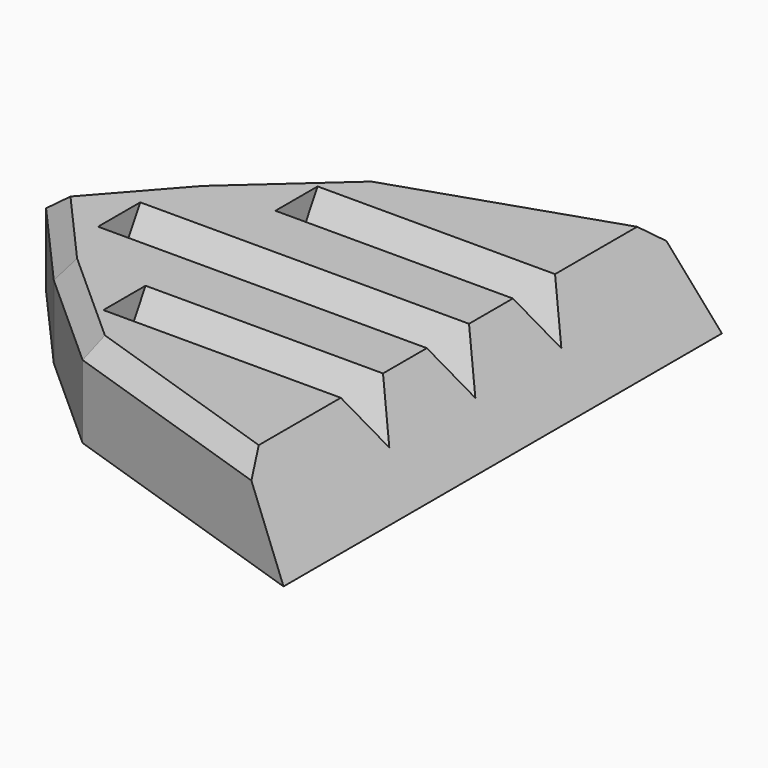
from build123d import *

# Parameters (mm, degrees)
F1_DEPTH    = 12.7
F3_DEPTH    = 40.64
F4_DEPTH    = 53.34
F5_T1_DEPTH = 85.1725092407
F5_T3_DEPTH = 73.3110318687
F5_T5_DEPTH = 73.3110318687
F5_T7_DEPTH = 85.1725092407
F6_SIZE     = 2.54


# Not quite as in the source:
# - a fillet or chamfer that OpenCascade refuses, or shapes differently, is made with other operations: its cross-section is extruded or revolved along the edge and cut away or added


with BuildPart() as f1:
    # F0 (on Top) → F1 (new body)
    with BuildSketch(Plane.XY):
        Polygon((0, -38.1), (0, 38.1), (-38.1, 25.4), (-52.2708785332, 12.7), (-63.5, 0), (-52.2708785332, -12.7), (-38.1, -25.4), align=None)
    extrude(amount=F1_DEPTH)

    # F2 (on face) → F3 (cut)
    with BuildSketch(Plane.YZ):
        Polygon((-14.9523484187, 6.35), (-11.2861742094, 12.7), (-18.6185226281, 12.7), align=None)
        Polygon((18.6185226281, 12.7), (11.2861742094, 12.7), (14.9523484187, 6.35), align=None)
    extrude(amount=-F3_DEPTH, mode=Mode.SUBTRACT)

    # F2 (on face) → F4 (cut)
    with BuildSketch(Plane.YZ):
        Polygon((3.6661742094, 12.7), (-3.6661742094, 12.7), (0, 6.35), align=None)
    extrude(amount=-F4_DEPTH, mode=Mode.SUBTRACT)

    # F5: chamfer of 7.62 x 12.7 on 4 edges, made by hand

    # F5_s2 → F5_t1 (cut)
    with BuildSketch(Plane.XZ.offset(-14.2269933063)):
        Polygon((-7.62, 12.7), (0, 0), (0, 12.7), align=None)
    extrude(amount=F5_T1_DEPTH, mode=Mode.SUBTRACT)

    # F5_s4 → F5_t3 (cut)
    with BuildSketch(Plane.XZ.offset(-29.179341725)):
        Polygon((-7.62, 12.7), (0, 0), (0, 12.7), align=None)
    extrude(amount=F5_T3_DEPTH, mode=Mode.SUBTRACT)

    # F5_s6 → F5_t5 (cut)
    with BuildSketch(Plane.XZ.offset(-44.1316901437)):
        Polygon((-7.62, 12.7), (0, 0), (0, 12.7), align=None)
    extrude(amount=F5_T5_DEPTH, mode=Mode.SUBTRACT)

    # F5_s8 → F5_t7 (cut)
    with BuildSketch(Plane.XZ.offset(-70.9455159344)):
        Polygon((-7.62, 12.7), (0, 0), (0, 12.7), align=None)
    extrude(amount=F5_T7_DEPTH, mode=Mode.SUBTRACT)

    # F6
    f6_edges = [f1.edges().sort_by_distance(p)[0] for p in [
        (-22.86, -30.48, 12.7),
        (-45.185439, -19.05, 12.7),
        (-57.885439, -6.35, 12.7),
        (-57.885439, 6.35, 12.7),
        (-45.185439, 19.05, 12.7),
        (-22.86, 30.48, 12.7),
    ]]
    chamfer(f6_edges, length=F6_SIZE)


solid = f1.part
